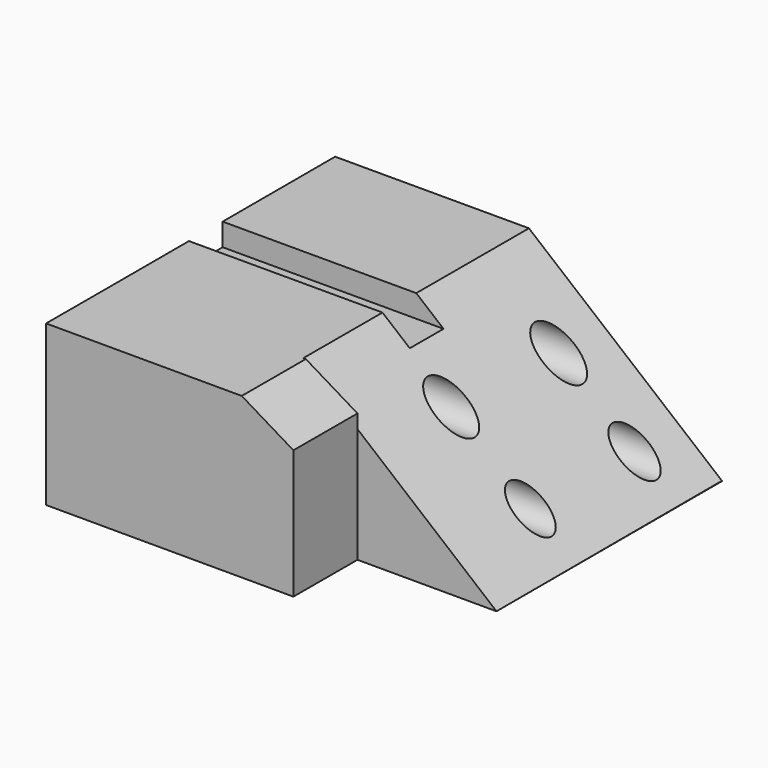
from build123d import *

# Parameters (mm, degrees)
F1_DEPTH  = 50.8
F3_DEPTH  = 0.189480841
F4_DEPTH  = 89.7186418795
F5_W      = 13.382118661
F5_H      = 7.166751343
F6_DEPTH  = 122.8903324733
F7_W      = 78.6715284359
F7_H      = 50.8
F8_DEPTH  = 25.4
F10_DEPTH = 25.4
F11_R     = 6.2312707334
F12_DEPTH = 122.8903324733
F13_R     = 6.1393781486
F14_DEPTH = 122.8903324733
F15_R     = 5.7324119576
F16_DEPTH = 122.8903324733
F17_R     = 5.5689542342
F18_DEPTH = 122.8903324733


with BuildPart() as f1:
    # F0 (on Top) → F1 (new body)
    with BuildSketch(Plane.XY):
        Polygon((-62.2928291559, 52.9630370438), (-62.2928291559, -36.376748234), (60.5965033174, -36.5652292967), (60.5965033174, 52.9630370438), align=None)
    extrude(amount=F1_DEPTH)

    # F2 (on face) → F3 (join, through all)
    with BuildSketch(Plane(origin=(-0.0559391088, -36.4722038357, 0), x_dir=(0.9999988238, -0.0015337445, 0), z_dir=(-0.0015337445, -0.9999988238, 0))):
        Polygon((60.6525137648, 50.8), (-0.7922247423, 50.8), (60.6525137648, 0), align=None)
    extrude(amount=F3_DEPTH)

    # F4 (cut, through all): a face of the model
    f4_faces = [f1.faces().sort_by_distance(p)[0] for p in [
        (40.1146572899, -36.7232964043, 33.8666666667),
    ]]
    extrude(f4_faces, amount=-F4_DEPTH, mode=Mode.SUBTRACT)

    # F5 (on face) → F6 (cut, through all)
    with BuildSketch(Plane(origin=(-62.2928291559, 0, 0), x_dir=(0, -1, 0), z_dir=(-1, 0, 0))):
        with Locations((-1.6020850744, 47.2166243285)):
            Rectangle(F5_W, F5_H)
    extrude(amount=-F6_DEPTH, mode=Mode.SUBTRACT)

    # F7 (on face) → F8 (join)
    with BuildSketch(Plane(origin=(-0.0559391088, -36.4722038357, 0), x_dir=(0.9999988238, -0.0015337445, 0), z_dir=(-0.0015337445, -0.9999988238, 0))):
        with Locations((-22.9011990315, 25.4)):
            Rectangle(F7_W, F7_H)
    extrude(amount=F8_DEPTH)

    # F9 (on face) → F10 (cut)
    with BuildSketch(Plane(origin=(-0.0948962197, -61.8721739606, 0), x_dir=(0.9999988238, -0.0015337445, 0), z_dir=(-0.0015337445, -0.9999988238, 0))):
        Polygon((16.4345651865, 50.8), (0, 50.8), (16.4345651865, 40.9449264407), align=None)
    extrude(amount=-F10_DEPTH, mode=Mode.SUBTRACT)

    # F11 (on face) → F12 (cut, through all)
    with BuildSketch(Plane(origin=(-62.2928291559, 0, 0), x_dir=(0, -1, 0), z_dir=(-1, 0, 0))):
        with Locations((-34.8689034581, 31.0050528497)):
            Circle(F11_R)
    extrude(amount=-F12_DEPTH, mode=Mode.SUBTRACT)

    # F13 (on face) → F14 (cut, through all)
    with BuildSketch(Plane(origin=(-62.2928291559, 0, 0), x_dir=(0, -1, 0), z_dir=(-1, 0, 0))):
        with Locations((6.031378638, 32.1359373629)):
            Circle(F13_R)
    extrude(amount=-F14_DEPTH, mode=Mode.SUBTRACT)

    # F15 (on face) → F16 (cut, through all)
    with BuildSketch(Plane(origin=(-62.2928291559, 0, 0), x_dir=(0, -1, 0), z_dir=(-1, 0, 0))):
        with Locations((-35.0573845208, 11.2145934254)):
            Circle(F15_R)
    extrude(amount=-F16_DEPTH, mode=Mode.SUBTRACT)

    # F17 (on face) → F18 (cut, through all)
    with BuildSketch(Plane(origin=(-62.2928291559, 0, 0), x_dir=(0, -1, 0), z_dir=(-1, 0, 0))):
        with Locations((5.6544179097, 11.5915555507)):
            Circle(F17_R)
    extrude(amount=-F18_DEPTH, mode=Mode.SUBTRACT)


solid = f1.part
